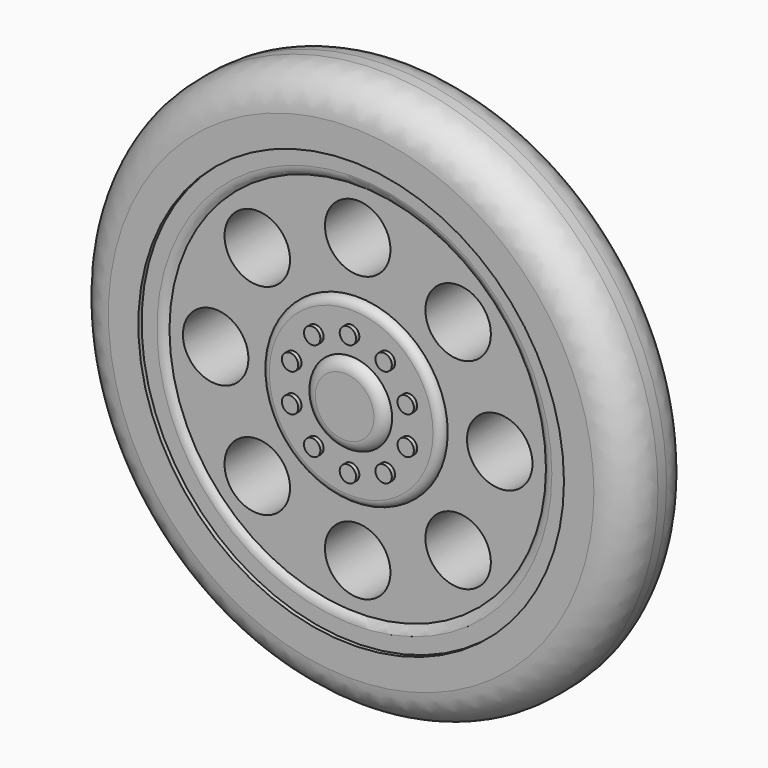
from build123d import *

# Parameters (mm, degrees)
F0_R      = 17
F1_DEPTH  = 4
F2_R      = 2
F3_DEPTH  = 25
F5_R      = 5.5
F6_DEPTH  = 0.5
F7_R      = 2.5
F8_DEPTH  = 0.5
F9_R      = 0.5
F10_DEPTH = 0.25
F11_R     = 17
F11_R_2   = 13
F12_DEPTH = 0.5
F13_R     = 13
F13_R_2   = 11.5
F14_DEPTH = 0.25
F4_R      = 17
F4_R_2    = 13
F15_DEPTH = 0.5
F16_R     = 13
F16_R_2   = 11.5
F17_DEPTH = 0.25
F18_R     = 2.1727922061
F19_R     = 3
F20_DEPTH = 8
F21_R     = 1.5
F22_DEPTH = 9
F24_R     = 0.49999


# Not quite as in the source:
# - a fillet or chamfer that OpenCascade refuses, or shapes differently, is made with other operations: its cross-section is extruded or revolved along the edge and cut away or added
# - a fillet or chamfer is up to 0.001 mm smaller than in the source, because OpenCascade refuses the exact size


with BuildPart() as f1:
    # F0 (on Front) → F1 (new body)
    with BuildSketch(Plane.XZ):
        Circle(F0_R)
    extrude(amount=F1_DEPTH)

    # F2 (on face) → F3 (cut)
    with BuildSketch(Plane.XZ.offset(4)):
        with Locations((0, 8.6762513965)):
            Circle(F2_R)
        with Locations((-6.1350361978, 6.1350361978)):
            Circle(F2_R)
        with Locations((-8.6762513965, 0)):
            Circle(F2_R)
        with Locations((-6.1350361978, -6.1350361978)):
            Circle(F2_R)
        with Locations((0, -8.6762513965)):
            Circle(F2_R)
        with Locations((6.1350361978, -6.1350361978)):
            Circle(F2_R)
        with Locations((8.6762513965, 0)):
            Circle(F2_R)
        with Locations((6.1350361978, 6.1350361978)):
            Circle(F2_R)
    extrude(amount=-F3_DEPTH, mode=Mode.SUBTRACT)

    # F5 (on face) → F6 (join)
    with BuildSketch(Plane.XZ.offset(4)):
        Circle(F5_R)
    extrude(amount=F6_DEPTH)

    # F7 (on face) → F8 (join)
    with BuildSketch(Plane.XZ.offset(4.5)):
        Circle(F7_R)
    extrude(amount=F8_DEPTH)

    # F9 (on face) → F10 (join)
    with BuildSketch(Plane.XZ.offset(4.5)):
        with Locations((0, 3.7141400389)):
            Circle(F9_R)
        with Locations((-2.1831167398, 3.004802411)):
            Circle(F9_R)
        with Locations((-3.5323570865, 1.1477323915)):
            Circle(F9_R)
        with Locations((-3.5323570865, -1.1477323915)):
            Circle(F9_R)
        with Locations((-2.1831167398, -3.004802411)):
            Circle(F9_R)
        with Locations((0, -3.7141400389)):
            Circle(F9_R)
        with Locations((2.1831167398, -3.004802411)):
            Circle(F9_R)
        with Locations((3.5323570865, -1.1477323915)):
            Circle(F9_R)
        with Locations((3.5323570865, 1.1477323915)):
            Circle(F9_R)
        with Locations((2.1831167398, 3.004802411)):
            Circle(F9_R)
    extrude(amount=F10_DEPTH)

    # F11 (on face) → F12 (join)
    with BuildSketch(Plane(origin=(0, 0, 0), x_dir=(-1, 0, 0), z_dir=(0, 1, 0))):
        Circle(F11_R)
        Circle(F11_R_2, mode=Mode.SUBTRACT)
    extrude(amount=F12_DEPTH)

    # F13 (on face) → F14 (join)
    with BuildSketch(Plane(origin=(0, 0, 0), x_dir=(-1, 0, 0), z_dir=(0, 1, 0))):
        Circle(F13_R)
        Circle(F13_R_2, mode=Mode.SUBTRACT)
    extrude(amount=F14_DEPTH)

    # F4 (on face) → F15 (join)
    with BuildSketch(Plane.XZ.offset(4)):
        Circle(F4_R)
        Circle(F4_R_2, mode=Mode.SUBTRACT)
    extrude(amount=F15_DEPTH)

    # F16 (on face) → F17 (join)
    with BuildSketch(Plane.XZ.offset(4)):
        Circle(F16_R)
        Circle(F16_R_2, mode=Mode.SUBTRACT)
    extrude(amount=F17_DEPTH)

    # F18
    f18_edges = [f1.edges().sort_by_distance(p)[0] for p in [
        (-17, -4.5, 0),
        (17, -2, 0),
        (-17, -4, 0),
        (0, 0, 17),
        (0, 0, -17),
        (-17, 0.25, 0),
        (17, 0.5, 0),
        (17, -4.25, 0),
    ]]
    fillet(f18_edges, radius=F18_R)

    # F19 (on face) → F20 (join)
    with BuildSketch(Plane(origin=(0, 0, 0), x_dir=(-1, 0, 0), z_dir=(0, 1, 0))):
        Circle(F19_R)
    extrude(amount=F20_DEPTH)

    # F21 (on face) → F22 (cut)
    with BuildSketch(Plane(origin=(0, 8, 0), x_dir=(-1, 0, 0), z_dir=(0, 1, 0))):
        Circle(F21_R)
    extrude(amount=-F22_DEPTH, mode=Mode.SUBTRACT)

    # F23: fillet of radius 0.75 on 1 edges, made by hand

    # F23_s1 → F23_t2 (revolve, cut)
    with BuildSketch(Plane.XY):
        with BuildLine():
            ThreePointArc((2.5, -4.5), (2.2259059207, -4.8623724357), (1.7928932188, -5))
            Line((1.7928932188, -5), (2.5, -5))
            Line((2.5, -5), (2.5, -4.5))
        make_face()
    revolve(axis=Axis((0, -5, 0), (0, -1, 0)), mode=Mode.SUBTRACT)

    # F24 (radius 0.5 in the source; OpenCascade refuses exactly that, so slightly less here)
    f24_edges = [f1.edges().sort_by_distance(p)[0] for p in [
        (-5.5, -4.5, 0),
    ]]
    fillet(f24_edges, radius=F24_R)

    # F25: fillet of radius 0.75 on 1 edges, made by hand

    # F25_s1 → F25_t2 (revolve, cut)
    with BuildSketch(Plane.XY):
        with BuildLine():
            ThreePointArc((11.5, -4), (11.7528307765, -4.1846531969), (12.0590169944, -4.25))
            Line((12.0590169944, -4.25), (11.5, -4.25))
            Line((11.5, -4.25), (11.5, -4))
        make_face()
    revolve(axis=Axis((0, -4.25, 0), (0, -1, 0)), mode=Mode.SUBTRACT)


solid = f1.part
